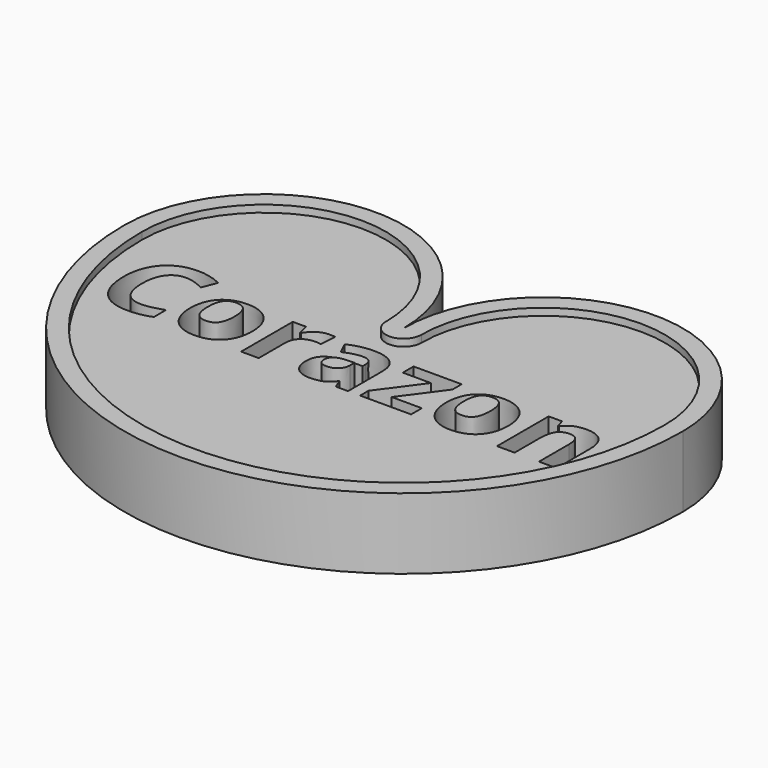
from build123d import *

# Parameters (mm, degrees)
F1_DEPTH     = 25.4
F2_TEXT_SIZE = 42.3333333333
F3_DEPTH     = 25.4
F5_DEPTH     = 2.54


# Not quite as in the source:
# - Text() gives the source's letters only with a copy of the font that has no kerning and outlines rounded to 1/6400 em; it was checked with that copy


with BuildPart() as f1:
    # F0 (on Top) → F1 (new body)
    with BuildSketch(Plane.XY):
        with BuildLine():
            ThreePointArc((100, 50), (50, 100), (0, 50))
            ThreePointArc((0, 50), (-50, 100), (-100, 50))
            ThreePointArc((-100, 50), (0, -50), (100, 50))
        make_face()
    extrude(amount=F1_DEPTH)

    # F2 (on face) → F3 (cut)
    with BuildSketch(Plane.XY.offset(25.4)):
        with Locations((-86.17526512, 14.3586324721)):
            Text('Corazon', F2_TEXT_SIZE, font='Open Sans', font_style=FontStyle.BOLD, text_align=(TextAlign.LEFT, TextAlign.BOTTOM))
    extrude(amount=-F3_DEPTH, mode=Mode.SUBTRACT)

    # F4 (on face) → F5 (cut)
    with BuildSketch(Plane.XY.offset(25.4)):
        with BuildLine():
            ThreePointArc((-6.35, 50), (-50, 93.65), (-93.65, 50))
            ThreePointArc((-93.65, 50), (0, -43.65), (93.65, 50))
            ThreePointArc((93.65, 50), (50, 93.65), (6.35, 50))
            ThreePointArc((6.35, 50), (0, 43.65), (-6.35, 50))
        make_face()
        with BuildLine():
            add(Edge.make_bspline(
                [(-61.82698387, 20.8673824721), (-66.35135887, 19.2798824721), (-77.1199005366, 19.2798824721), (-77.1199005366, 34.2420699721), (-73.1511505366, 39.6792574721), (-67.87932762, 39.6792574721), (-64.4529734533, 38.4820178888), (-62.7530255366, 37.6750387221)],
                knots=[0, 0, 0, 1, 3.3846153846, 4.530104712, 5.6755940395, 6.1991266388, 6.7226592382, 6.7226592382, 6.7226592382], degree=2))
            Line((-61.82698387, 20.8673824721), (-61.82698387, 15.4963408054))
            add(Edge.make_bspline(
                [(-60.6892755366, 42.8873303888), (-65.1342755366, 45.0106116388), (-73.85229637, 45.0106116388), (-80.28167137, 41.2336845554), (-83.71464012, 34.1428512221), (-83.71464012, 21.9455595554), (-76.72964012, 13.9419137221), (-65.5443797033, 13.9419137221), (-61.82698387, 15.4963408054)],
                knots=[0, 0, 0, 1, 1.9819548872, 2.9639097744, 3.9458646617, 5.5034957661, 7.0611268705, 8.1453756031, 8.1453756031, 8.1453756031], degree=2))
            Line((-60.6892755366, 42.8873303888), (-62.7530255366, 37.6750387221))
        make_face(mode=Mode.SUBTRACT)
        with BuildLine():
            add(Edge.make_bspline(
                [(-34.8924005366, 25.9539970554), (-34.8924005366, 29.5920178888), (-37.61760887, 35.0093616388), (-42.7042234533, 37.8999345554), (-51.38917137, 37.8999345554), (-57.2959942866, 31.6160803888), (-57.2959942866, 22.3159762221), (-54.5707859533, 16.8589449721), (-49.48417137, 13.9419137221), (-40.8455255366, 13.9419137221), (-34.8924005366, 20.3117574721), (-34.8924005366, 25.9539970554)],
                knots=[0, 0, 0, 1, 2, 3, 4.6103379722, 6.2206759443, 7.2553557162, 8.290035488, 9.3247152598, 10.9765002634, 12.6282852669, 12.6282852669, 12.6282852669], degree=2))
        make_face(mode=Mode.SUBTRACT)
        with BuildLine():
            add(Edge.make_bspline(
                [(-14.6517755366, 37.7147262221), (-15.4984422033, 37.8999345554), (-18.9314109533, 37.8999345554), (-22.5892755366, 35.5252991388), (-23.66745262, 33.5806116388)],
                knots=[0, 0, 0, 1, 2.675257732, 4.3505154639, 4.3505154639, 4.3505154639], degree=2))
            Line((-14.6517755366, 37.7147262221), (-15.1280255366, 31.8079033054))
            add(Edge.make_bspline(
                [(-23.3764109533, 26.1193616388), (-23.3764109533, 28.9107158054), (-20.0029734533, 32.0129553888), (-15.8953172033, 32.0129553888), (-15.1280255366, 31.8079033054)],
                knots=[0, 0, 0, 1, 2, 2.3618421053, 2.3618421053, 2.3618421053], degree=2))
            Line((-23.3764109533, 26.1193616388), (-23.3764109533, 14.3586324721))
            Line((-23.3764109533, 14.3586324721), (-29.68010887, 14.3586324721))
            Line((-29.68010887, 14.3586324721), (-29.68010887, 37.4699866388))
            Line((-29.68010887, 37.4699866388), (-24.9043797033, 37.4699866388))
            Line((-24.9043797033, 37.4699866388), (-23.9717234533, 33.5806116388))
            Line((-23.9717234533, 33.5806116388), (-23.66745262, 33.5806116388))
        make_face(mode=Mode.SUBTRACT)
        with BuildLine():
            Line((8.61832863, 14.3586324721), (4.2196307134, 14.3586324721))
            Line((4.2196307134, 14.3586324721), (2.9959327967, 17.5005595554))
            Line((2.9959327967, 17.5005595554), (2.8305682134, 17.5005595554))
            add(Edge.make_bspline(
                [(-1.6541192866, 28.6196741388), (-6.83995262, 28.4344658054), (-11.9860984533, 24.9419658054), (-11.9860984533, 17.7519137221), (-8.1628692866, 13.9419137221), (-2.1303692866, 13.9419137221), (1.2430682134, 15.4963408054), (2.8305682134, 17.5005595554)],
                knots=[0, 0, 0, 1, 2, 2.9550359712, 3.9100719424, 4.6866320065, 5.4631920706, 5.4631920706, 5.4631920706], degree=2))
            Line((-1.6541192866, 28.6196741388), (2.3609327967, 28.7453512221))
            Line((2.3609327967, 28.7453512221), (2.3609327967, 29.7573824721))
            add(Edge.make_bspline(
                [(-7.75276512, 31.5962366388), (-4.0089109533, 33.2697262221), (2.3609327967, 33.2697262221), (2.3609327967, 29.7573824721)],
                knots=[0, 0, 0, 1, 2.2983293556, 2.2983293556, 2.2983293556], degree=2))
            Line((-7.75276512, 31.5962366388), (-9.83635887, 35.8560283054))
            add(Edge.make_bspline(
                [(8.61832863, 29.7573824721), (8.61832863, 33.8914970554), (3.65739113, 37.9462366388), (-5.84776512, 37.9462366388), (-9.83635887, 35.8560283054)],
                knots=[0, 0, 0, 1, 2, 3.0440967283, 3.0440967283, 3.0440967283], degree=2))
            Line((8.61832863, 29.7573824721), (8.61832863, 14.3586324721))
        make_face(mode=Mode.SUBTRACT)
        Polygon((31.1939015467, 19.1740491388), (31.1939015467, 14.3586324721), (12.94426613, 14.3586324721), (12.94426613, 18.0826428888), (23.6532765467, 32.6545699721), (13.5858807134, 32.6545699721), (13.5858807134, 37.4699866388), (30.82348488, 37.4699866388), (30.82348488, 33.3755595554), (20.40551613, 19.1740491388), align=None, mode=Mode.SUBTRACT)
        with BuildLine():
            add(Edge.make_bspline(
                [(56.7658807134, 25.9539970554), (56.7658807134, 29.5920178888), (54.04067238, 35.0093616388), (48.9540577967, 37.8999345554), (40.26910988, 37.8999345554), (34.3622869634, 31.6160803888), (34.3622869634, 22.3159762221), (37.0874952967, 16.8589449721), (42.17410988, 13.9419137221), (50.8127557134, 13.9419137221), (56.7658807134, 20.3117574721), (56.7658807134, 25.9539970554)],
                knots=[0, 0, 0, 1, 2, 3, 4.6103379722, 6.2206759443, 7.2553557162, 8.290035488, 9.3247152598, 10.9765002634, 12.6282852669, 12.6282852669, 12.6282852669], degree=2))
        make_face(mode=Mode.SUBTRACT)
        with BuildLine():
            Line((83.31020363, 29.4266533054), (83.31020363, 14.3586324721))
            Line((83.31020363, 14.3586324721), (77.0065057134, 14.3586324721))
            Line((77.0065057134, 14.3586324721), (77.0065057134, 27.8589970554))
            add(Edge.make_bspline(
                [(68.2818702967, 25.2330074721), (68.2818702967, 29.3274345554), (70.6366619634, 32.8596220554), (75.2271827967, 32.8596220554), (77.0065057134, 30.3593095554), (77.0065057134, 27.8589970554)],
                knots=[0, 0, 0, 1, 2, 2.735, 3.47, 3.47, 3.47], degree=2))
            Line((68.2818702967, 25.2330074721), (68.2818702967, 14.3586324721))
            Line((68.2818702967, 14.3586324721), (61.97817238, 14.3586324721))
            Line((61.97817238, 14.3586324721), (61.97817238, 37.4699866388))
            Line((61.97817238, 37.4699866388), (66.7935890467, 37.4699866388))
            Line((66.7935890467, 37.4699866388), (67.6402557134, 34.5132678888))
            Line((67.6402557134, 34.5132678888), (67.99082863, 34.5132678888))
            add(Edge.make_bspline(
                [(83.31020363, 29.4266533054), (83.31020363, 33.5409241388), (79.1364015467, 37.8999345554), (72.7467140467, 37.8999345554), (69.0491619634, 36.1867574721), (67.99082863, 34.5132678888)],
                knots=[0, 0, 0, 1, 2, 2.5836065574, 3.1672131148, 3.1672131148, 3.1672131148], degree=2))
        make_face(mode=Mode.SUBTRACT)
    extrude(amount=-F5_DEPTH, mode=Mode.SUBTRACT)


solid = f1.part
